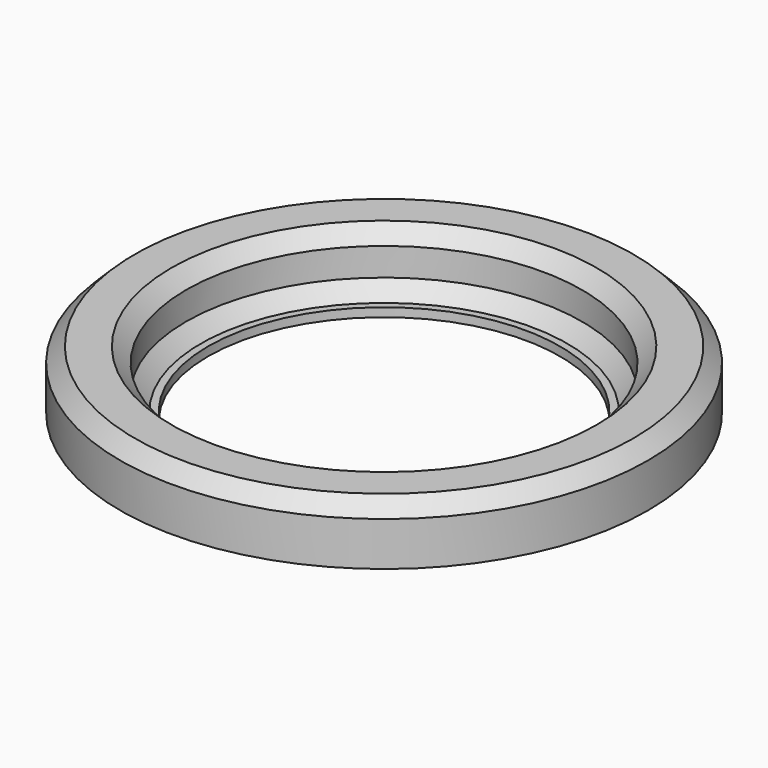
from build123d import *

# Parameters (mm, degrees)
F0_R          = 18
F0_R_2        = 13.5
F1_DEPTH      = 4
F0_R_3        = 12
F2_DEPTH      = 0.5
F2_DEPTH_BACK = 0.1
F3_SIZE       = 1
F4_SIZE       = 1


with BuildPart() as f1:
    # F0 (on Top) → F1 (new body)
    with BuildSketch(Plane.XY):
        Circle(F0_R)
        Circle(F0_R_2, mode=Mode.SUBTRACT)
    extrude(amount=F1_DEPTH)

    # F0 (on Top) → F2 (join, two sides)
    with BuildSketch(Plane.XY) as f2_sk:
        Circle(F0_R_2)
        Circle(F0_R_3, mode=Mode.SUBTRACT)
    extrude(amount=-F2_DEPTH)
    extrude(f2_sk.sketch, amount=F2_DEPTH_BACK)

    # F3
    f3_edges = [f1.edges().sort_by_distance(p)[0] for p in [
        (-13.5, 0, 0.1),
    ]]
    chamfer(f3_edges, length=F3_SIZE)

    # F4
    f4_edges = [f1.edges().sort_by_distance(p)[0] for p in [
        (-18, 0, 4),
        (-13.5, 0, 4),
    ]]
    chamfer(f4_edges, length=F4_SIZE)


solid = f1.part
